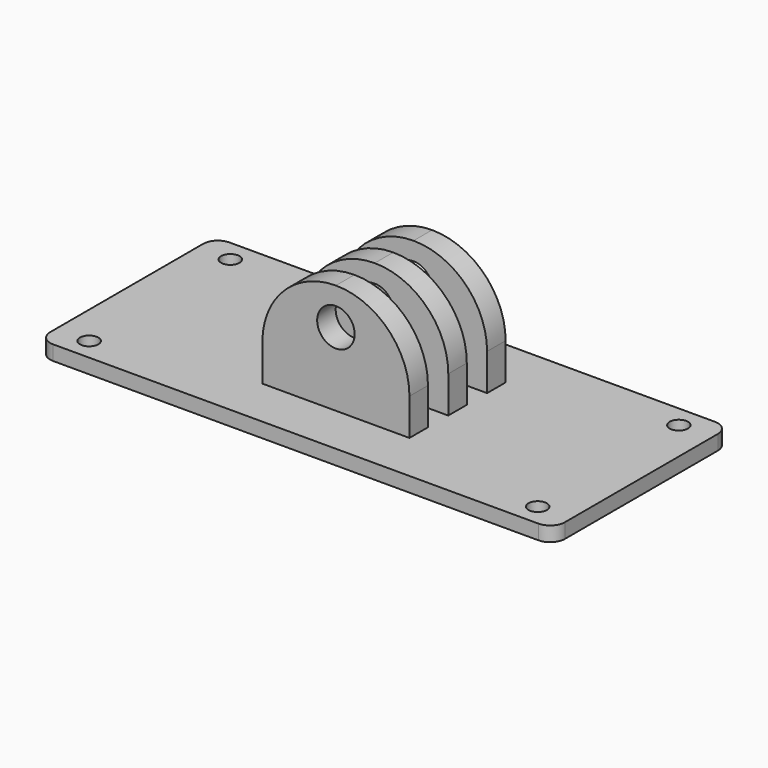
from build123d import *

# Parameters (mm, degrees)
F0_R     = 1.25
F1_DEPTH = 2
F2_W     = 20
F2_H     = 3.15
F3_DEPTH = 15
F4_R     = 9.99999
F5_R     = 2.55
F6_DEPTH = 25


# Not quite as in the source:
# - a fillet or chamfer is up to 0.001 mm smaller than in the source, because OpenCascade refuses the exact size


with BuildPart() as f1:
    # F0 (on Top) → F1 (new body)
    with BuildSketch(Plane.XY):
        with BuildLine():
            Line((-33, -15), (33, -15))
            ThreePointArc((33, -15), (34.4142135624, -14.4142135624), (35, -13))
            Line((35, -13), (35, 13))
            ThreePointArc((35, 13), (34.4142135624, 14.4142135624), (33, 15))
            Line((33, 15), (-33, 15))
            ThreePointArc((-33, 15), (-34.4142135624, 14.4142135624), (-35, 13))
            Line((-35, 13), (-35, -13))
            ThreePointArc((-35, -13), (-34.4142135624, -14.4142135624), (-33, -15))
        make_face()
        with Locations((-30.5, -12)):
            Circle(F0_R, mode=Mode.SUBTRACT)
        with Locations((30.5, -12)):
            Circle(F0_R, mode=Mode.SUBTRACT)
        with Locations((-30.5, 12)):
            Circle(F0_R, mode=Mode.SUBTRACT)
        with Locations((30.5, 12)):
            Circle(F0_R, mode=Mode.SUBTRACT)
    extrude(amount=F1_DEPTH)

    # F2 (on face) → F3 (join)
    with BuildSketch(Plane.XY.offset(2)):
        Rectangle(F2_W, F2_H)
        with Locations((0, 6.6)):
            Rectangle(F2_W, F2_H)
        with Locations((0, -6.6)):
            Rectangle(F2_W, F2_H)
    extrude(amount=F3_DEPTH)

    # F4 (radius 10 in the source; OpenCascade refuses exactly that, so slightly less here)
    f4_edges = [f1.edges().sort_by_distance(p)[0] for p in [
        (-10, -6.6, 17),
        (10, -6.6, 17),
        (10, 0, 17),
        (-10, 0, 17),
        (-10, 6.6, 17),
        (10, 6.6, 17),
    ]]
    fillet(f4_edges, radius=F4_R)

    # F5 (on face) → F6 (cut)
    with BuildSketch(Plane.XZ.offset(8.175)):
        with Locations((0, 12)):
            Circle(F5_R)
    extrude(amount=-F6_DEPTH, mode=Mode.SUBTRACT)


solid = f1.part
